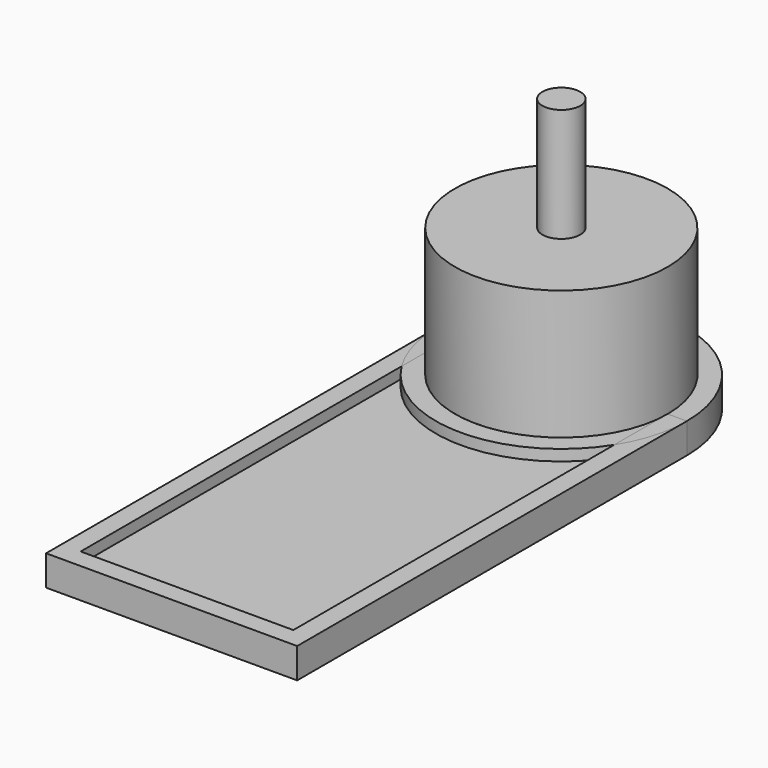
from build123d import *
from build123d import SkipClean  # not in build123d's __all__

# Parameters (mm, degrees)
F0_R     = 14.05
F1_DEPTH = 17.1
F2_R     = 2.5
F3_DEPTH = 15
F5_DEPTH = 4
F6_T     = -2.54
F7_DEPTH = 2.54


with BuildPart() as f1:
    # F0 (on Top) → F1 (new body)
    with BuildSketch(Plane.XY):
        Circle(F0_R)
    extrude(amount=F1_DEPTH)

    # F2 (on face) → F3 (join)
    with BuildSketch(Plane.XY.offset(17.1)):
        Circle(F2_R)
    extrude(amount=F3_DEPTH)


with BuildPart() as f5:
    # F4 (on face) → F5 (new body)
    with BuildSketch(Plane(origin=(0, 0, 0), x_dir=(1, 0, 0), z_dir=(0, 0, -1))):
        with BuildLine():
            Line((14.05, 0), (16.59, 0))
            ThreePointArc((16.59, 0), (0, 16.59), (-16.59, 0))
            Line((-16.59, 0), (-14.05, 0))
            ThreePointArc((-14.05, 0), (0, 14.05), (14.05, 0))
        make_face()
        with BuildLine():
            ThreePointArc((-16.59, 0), (0, -16.59), (16.59, 0))
            Line((16.59, 0), (14.05, 0))
            ThreePointArc((14.05, 0), (0, -14.05), (-14.05, 0))
            Line((-14.05, 0), (-16.59, 0))
        make_face()
        with BuildLine():
            ThreePointArc((-16.59, 0), (0, 16.59), (16.59, 0))
            Line((16.59, 0), (16.59, 64.369417727))
            Line((16.59, 64.369417727), (0, 64.369417727))
            Line((0, 64.369417727), (-16.59, 64.369417727))
            Line((-16.59, 64.369417727), (-16.59, 0))
        make_face()
        with BuildLine():
            ThreePointArc((-14.05, 0), (0, -14.05), (14.05, 0))
            Line((14.05, 0), (0, 0))
            Line((0, 0), (-14.05, 0))
        make_face()
        with BuildLine():
            Line((0, 0), (14.05, 0))
            ThreePointArc((14.05, 0), (0, 14.05), (-14.05, 0))
            Line((-14.05, 0), (0, 0))
        make_face()
    extrude(amount=F5_DEPTH)

    # F6
    f6_openings = [f5.faces().sort_by_distance(p)[0] for p in [
        (0, -25.581259, 0),
    ]]
    offset(amount=F6_T, openings=f6_openings)

    # F4 (on face) → F7 (join)
    with BuildSketch(Plane(origin=(0, 0, 0), x_dir=(1, 0, 0), z_dir=(0, 0, -1))):
        with BuildLine():
            Line((14.05, 0), (16.59, 0))
            ThreePointArc((16.59, 0), (0, 16.59), (-16.59, 0))
            Line((-16.59, 0), (-14.05, 0))
            ThreePointArc((-14.05, 0), (0, 14.05), (14.05, 0))
        make_face()
    with SkipClean():  # cleaning this boolean's faces spoils the solid; the shape is the same uncleaned
        extrude(amount=F7_DEPTH)


solid = Compound([f1.part, f5.part])
